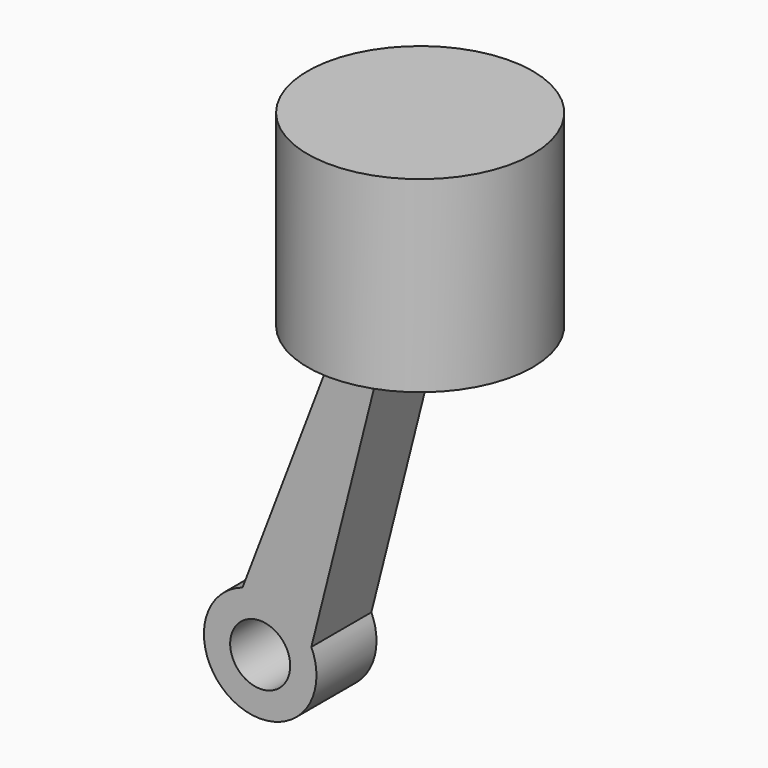
from build123d import *

# Parameters (mm, degrees)
F1_W          = 15
F1_H          = 25
F3_T          = -3
F4_DEPTH      = 12.0000001006
F4_DEPTH_BACK = 12.0000001006
F5_R          = 2.5
F6_DEPTH      = 5
F7_W          = 10
F7_H          = 7
F8_DEPTH      = 12
F8_DEPTH_BACK = 12
F9_R          = 2.5
F9_R_2        = 4
F10_DEPTH     = 5


with BuildPart() as f2:
    # F1 (on Front) → F2 (revolve)
    with BuildSketch(Plane.XZ):
        with Locations((7.5, 64.7015325446)):
            Rectangle(F1_W, F1_H)
    revolve(axis=Axis((0, 0, 62.2015325446), (0, 0, 1)))

    # F3
    f3_openings = [f2.faces().sort_by_distance(p)[0] for p in [
        (0, 0, 52.201533),
    ]]
    offset(amount=F3_T, openings=f3_openings)

    # F0 (on Front) → F4 (join, two sides)
    with BuildSketch(Plane.XZ) as f4_sk:
        with BuildLine():
            ThreePointArc((-5, 62.2015325446), (-4.0541927813, 59.2751831307), (-1.5745916432, 57.4559386769))
            ThreePointArc((-1.5745916432, 57.4559386769), (2.9263494138, 58.1473397632), (5, 62.2015325446))
            Line((5, 62.2015325446), (5, 70.2015325446))
            Line((5, 70.2015325446), (-5, 70.2015325446))
            Line((-5, 70.2015325446), (-5, 62.2015325446))
        make_face()
        with BuildLine():
            ThreePointArc((2.5, 62.2015325446), (1.4631747069, 60.1744361539), (-0.7872958216, 59.8287356107))
            ThreePointArc((-0.7872958216, 59.8287356107), (-1.4631747069, 64.2286289352), (2.5, 62.2015325446))
        make_face(mode=Mode.SUBTRACT)
    extrude(amount=-F4_DEPTH)
    extrude(f4_sk.sketch, amount=F4_DEPTH_BACK)

    # F5 (on Front) → F6 (cut, symmetric)
    with BuildSketch(Plane.XZ):
        with BuildLine():
            Line((5, 70.2015325446), (-5, 70.2015325446))
            Line((-5, 70.2015325446), (-5, 62.2015325446))
            ThreePointArc((-5, 62.2015325446), (0, 57.2015325446), (5, 62.2015325446))
            Line((5, 62.2015325446), (5, 70.2015325446))
        make_face()
        with Locations((0, 62.2015325446)):
            Circle(F5_R, mode=Mode.SUBTRACT)
    extrude(amount=F6_DEPTH, both=True, mode=Mode.SUBTRACT)

    # F7 (on Front) → F8 (join, two sides)
    with BuildSketch(Plane.XZ) as f8_sk:
        with Locations((0, 73.7015325446)):
            Rectangle(F7_W, F7_H)
    extrude(amount=F8_DEPTH)
    extrude(f8_sk.sketch, amount=-F8_DEPTH_BACK)


with BuildPart() as f10:
    # F9 (on Front) → F10 (new body, symmetric)
    with BuildSketch(Plane.XZ):
        with BuildLine():
            ThreePointArc((0, 54.7015325446), (5.3033008589, 56.8982316857), (7.5, 62.2015325446))
            ThreePointArc((7.5, 62.2015325446), (-3.232233047, 68.9692994975), (-4.7140452079, 56.3681992112))
            ThreePointArc((-4.7140452079, 56.3681992112), (-2.5, 55.1304647327), (0, 54.7015325446))
        make_face()
        with Locations((0, 62.2015325446)):
            Circle(F9_R, mode=Mode.SUBTRACT)
        with BuildLine():
            ThreePointArc((0, 54.7015325446), (-2.5, 55.1304647327), (-4.7140452079, 56.3681992112))
            Line((-4.7140452079, 56.3681992112), (-19.6716815341, 17.1219367709))
            ThreePointArc((-19.6716815341, 17.1219367709), (-14.325011455, 16.8758272226), (-10.5039119039, 13.1279412767))
            Line((-10.5039119039, 13.1279412767), (0, 54.7015325446))
        make_face()
        with BuildLine():
            ThreePointArc((-10.5039119039, 13.1279412767), (-14.325011455, 16.8758272226), (-19.6716815341, 17.1219367709))
            ThreePointArc((-19.6716815341, 17.1219367709), (-21.7146063371, 3.922015098), (-9.8205080757, 10))
            ThreePointArc((-9.8205080757, 10), (-9.9933506702, 11.6008636281), (-10.5039119039, 13.1279412767))
        make_face()
        with Locations((-17.3205080757, 10)):
            Circle(F9_R_2, mode=Mode.SUBTRACT)
    extrude(amount=F10_DEPTH, both=True)


solid = Compound([f2.part, f10.part])
